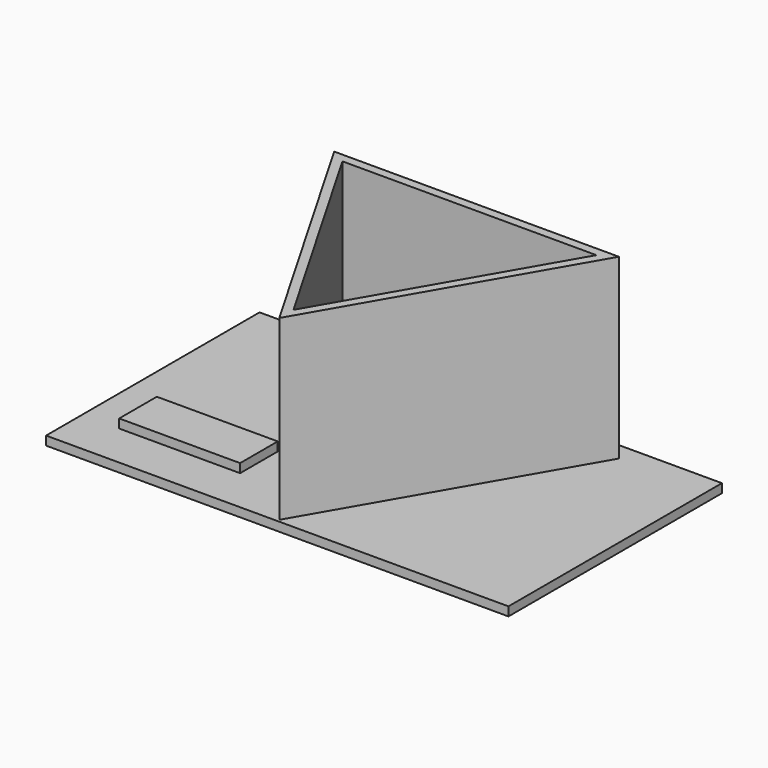
from build123d import *

# Parameters (mm, degrees)
F0_W        = 66.1063343287
F0_H        = 38.1483472884
F1_DEPTH    = 1.27
F3_DEPTH    = 25.4
F4_T        = 1.27
F4_T3_DEPTH = 43.2463343287
F4_T5_DEPTH = 43.2463343287
F4_T7_DEPTH = 43.2463343287
F5_W        = 17.286144197
F5_H        = 6.7250733264
F6_DEPTH    = 1.27


# Not quite as in the source:
# - a shell that OpenCascade refuses in one call is made with other operations: the cavity is built on its own and cut out


with BuildPart() as f1:
    # F0 (on Top) → F1 (new body)
    with BuildSketch(Plane.XY):
        Rectangle(F0_W, F0_H)
    extrude(amount=F1_DEPTH)

    # F2 (on face) → F3 (join)
    with BuildSketch(Plane.XY.offset(1.27)):
        Polygon((20.3531671643, 16.5341736442), (-20.3531671643, 16.5341736442), (0, -18.7185459794), align=None)
    extrude(amount=F3_DEPTH)

    # F4: shell of thickness 1.27, made by hand


with BuildPart() as f4_core1:
    # F4_t2: copy of F1
    add(f1.part)

    # the walls: a layer under each face that stays
    f4_faces = [f4_core1.faces().sort_by_distance(p)[0] for p in [
        (33.0531671643, 0, 0.635),
        (0, -19.0741736442, 0.635),
        (0, 19.0741736442, 0.635),
        (0, 0, 0),
        (-22.0354447762, -12.7161157628, 1.27),
        (-33.0531671643, 0, 0.635),
        (0, 16.5341736442, 13.97),
        (-10.1765835822, -1.0921861676, 13.97),
        (10.1765835822, -1.0921861676, 13.97),
    ]]
    thicken(f4_faces, amount=-F4_T, mode=Mode.SUBTRACT)

    # F4_s4 → F4_t3 (cut)
    with BuildSketch(Plane.YZ.offset(-21.6231671643)):
        Polygon((16.5468736442, 1.2827), (16.5341736442, 0), (15.2641736442, 0), (15.2641736442, 1.27), align=None)
    extrude(amount=F4_T3_DEPTH, mode=Mode.SUBTRACT)

    # F4_s6 → F4_t5 (cut)
    with BuildSketch(Plane(origin=(-12.8827989943, 22.3136624018, 0), x_dir=(0, 0, 1), z_dir=(0.5, -0.8660254038, 0))):
        Polygon((1.2827, 9.3719729897), (0, 9.3592729897), (0, 8.0892729897), (1.27, 8.0892729897), align=None)
    extrude(amount=F4_T5_DEPTH, mode=Mode.SUBTRACT)

    # F4_s8 → F4_t7 (cut)
    with BuildSketch(Plane(origin=(-8.74036817, -15.1387617473, 0), x_dir=(0, 0, 1), z_dir=(0.5, 0.8660254038, 0))):
        Polygon((1.2827, 9.3719729897), (0, 9.3592729897), (0, 8.0892729897), (1.27, 8.0892729897), align=None)
    extrude(amount=F4_T7_DEPTH, mode=Mode.SUBTRACT)


with BuildPart() as f1_1:
    add(f1.part)

    # what is left inside the walls is the cavity
    f4_cavity = [f4_core1.part.solids().sort_by_distance(p)[0] for p in [
        (-9.065733, -0.450836, 18.203333),
    ]]
    add(f4_cavity, mode=Mode.SUBTRACT)

    # F5 (on face) → F6 (join)
    with BuildSketch(Plane.XY.offset(1.27)):
        with Locations((-19.0954133868, -9.2882269528)):
            Rectangle(F5_W, F5_H)
    extrude(amount=F6_DEPTH)


solid = f1_1.part
